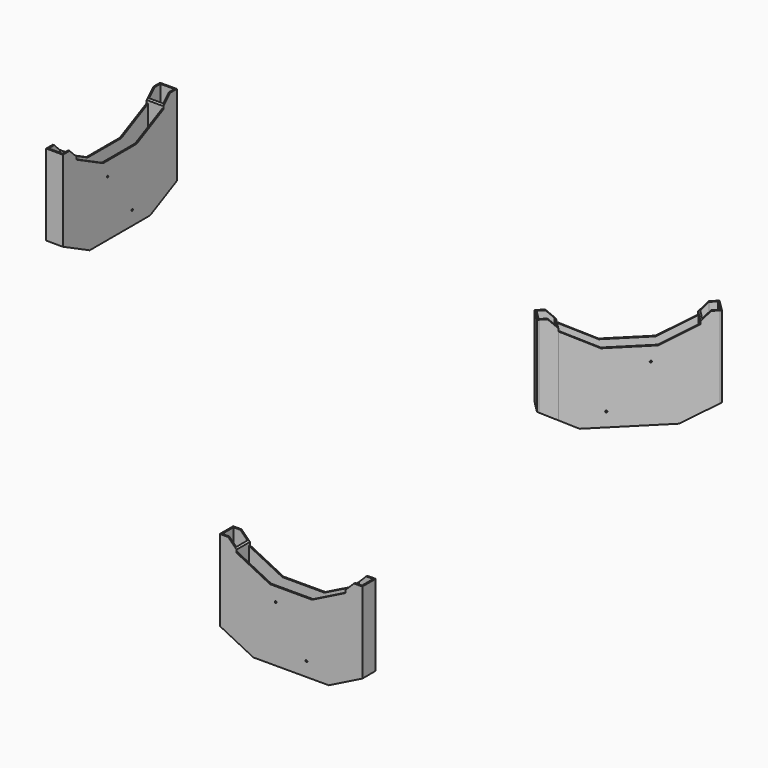
from build123d import *

# Parameters (mm, degrees)
F0_W          = 390
F0_H          = 5
F0_W_2        = 5
F0_H_2        = 50
F1_DEPTH      = 350
F0_H_3        = 390
F0_W_3        = 50
F2_R          = 3.25
F3_DEPTH      = 100
F4_R          = 3.25
F5_DEPTH      = 100
F6_R          = 3.25
F7_DEPTH      = 100
F8_T1_DEPTH   = 681.5589297088
F8_2_T1_DEPTH = 681.5589297088
F8_2_T3_DEPTH = 681.5589297088
F8_3_T1_DEPTH = 681.5589297088
F9_T1_DEPTH   = 214.3009792779
F9_2_T1_DEPTH = 214.300979278
F9_3_T1_DEPTH = 214.300979278


# Not quite as in the source:
# - a fillet or chamfer that OpenCascade refuses, or shapes differently, is made with other operations: its cross-section is extruded or revolved along the edge and cut away or added


with BuildPart() as f1:
    # F0 (on Top) → F1 (new body)
    with BuildSketch(Plane.XY):
        Polygon((90.3563703896, -1526.5155034513), (90.3563703896, -1531.5155034513), (480.3563703896, -1531.5155034513), (480.3563703896, -1526.5155034513), (460.3563703896, -1526.5155034513), (410.3563703896, -1526.5155034513), (160.3563703896, -1526.5155034513), (110.3563703896, -1526.5155034513), align=None)
        with Locations((285.3563703896, -1584.0155034513)):
            Rectangle(F0_W, F0_H)
        with Locations((87.8563703896, -1556.5155034513)):
            Rectangle(F0_W_2, F0_H_2)
        Polygon((30.3563703896, -1526.5155034513), (30.3563703896, -1531.5155034513), (35.3563703896, -1531.5155034513), (85.3563703896, -1531.5155034513), (90.3563703896, -1531.5155034513), (90.3563703896, -1526.5155034513), align=None)
        with Locations((32.8563703896, -1556.5155034513)):
            Rectangle(F0_W_2, F0_H_2)
        Polygon((30.3563703896, -1581.5155034513), (30.3563703896, -1586.5155034513), (90.3563703896, -1586.5155034513), (90.3563703896, -1581.5155034513), (85.3563703896, -1581.5155034513), (35.3563703896, -1581.5155034513), align=None)
        Polygon((480.3563703896, -1581.5155034513), (480.3563703896, -1586.5155034513), (540.3563703896, -1586.5155034513), (540.3563703896, -1581.5155034513), (535.3563703896, -1581.5155034513), (485.3563703896, -1581.5155034513), align=None)
        with Locations((482.8563703896, -1556.5155034513)):
            Rectangle(F0_W_2, F0_H_2)
        Polygon((480.3563703896, -1526.5155034513), (480.3563703896, -1531.5155034513), (485.3563703896, -1531.5155034513), (535.3563703896, -1531.5155034513), (540.3563703896, -1531.5155034513), (540.3563703896, -1526.5155034513), align=None)
        with Locations((537.8563703896, -1556.5155034513)):
            Rectangle(F0_W_2, F0_H_2)
    extrude(amount=F1_DEPTH)

    # F6 (on face) → F7 (cut)
    with BuildSketch(Plane.XZ.offset(1586.5155034513)):
        with Locations((230.3563703896, 200)):
            Circle(F6_R)
        with Locations((340.3563703896, 50)):
            Circle(F6_R)
        Polygon((480.3563703896, 350), (90.3563703896, 350), (90.3563703896, 310), (210.3563703896, 250), (360.3563703896, 250), (480.3563703896, 310), align=None)
    extrude(amount=-F7_DEPTH, mode=Mode.SUBTRACT)

    # F8: chamfer of 60 x 120 on 2 edges, made by hand

    # F8_s2 → F8_t1 (cut)
    with BuildSketch(Plane.XZ.offset(1215.7360385969)):
        Polygon((540.3563703896, 60), (420.3563703896, 0), (540.3563703896, 0), align=None)
        Polygon((30.3563703896, 60), (150.3563703896, 0), (30.3563703896, 0), align=None)
    extrude(amount=F8_T1_DEPTH, mode=Mode.SUBTRACT)

    # F9: chamfer of 30 on 2 edges, made by hand

    # F9_s2 → F9_t1 (cut)
    with BuildSketch(Plane.XZ.offset(1449.3650138123)):
        Polygon((510.3563703896, 350), (480.3563703896, 320), (480.3563703896, 350), align=None)
        Polygon((60.3563703896, 350), (90.3563703896, 320), (90.3563703896, 350), align=None)
    extrude(amount=F9_T1_DEPTH, mode=Mode.SUBTRACT)


with BuildPart() as f1b:
    # F0 (on Top) → F1, piece 2 (new body)
    with BuildSketch(Plane.XY):
        Polygon((215.6097792881, 288.056401427), (219.145313194, 284.520867521), (222.6808471, 288.056401427), (219.145313194, 291.5919353329), align=None)
        Polygon((197.9321097584, 270.3787318973), (201.4676436644, 266.8431979914), (219.145313194, 284.520867521), (215.6097792881, 288.056401427), align=None)
        Polygon((176.7189063228, 326.9472743922), (159.0412367932, 309.2696048626), (162.5767706991, 305.7340709566), (180.2544402288, 323.4117404863), align=None)
        Polygon((180.2544402288, 330.4828082982), (176.7189063228, 326.9472743922), (180.2544402288, 323.4117404863), (183.7899741347, 326.9472743922), align=None)
        Polygon((-44.251962798, 21.1235915291), (201.4676436644, 266.8431979914), (197.9321097584, 270.3787318973), (-47.7874967039, 24.659125435), align=None)
        Polygon((162.5767706991, 305.7340709566), (159.0412367932, 309.2696048626), (-86.6783696692, 63.5499984002), (-83.1428357632, 60.0144644943), align=None)
        Polygon((196.1643428055, 346.3927108749), (180.2544402288, 330.4828082982), (183.7899741347, 326.9472743922), (199.6998767114, 342.8571769689), align=None)
        Polygon((219.145313194, 291.5919353329), (222.6808471, 288.056401427), (238.5907496767, 303.9663040037), (235.0552157707, 307.5018379096), align=None)
        Polygon((-47.7874967039, 24.659125435), (-83.1428357632, 60.0144644943), (-86.6783696692, 56.4789305884), (-51.3230306098, 21.123591529), align=None)
        Polygon((-86.6783696692, 63.5499984002), (-125.5692426344, 24.659125435), (-122.0337087285, 21.123591529), (-86.6783696692, 56.4789305884), (-83.1428357632, 60.0144644943), align=None)
        Polygon((-122.0337087285, 21.123591529), (-125.5692426344, 17.5880576231), (-90.2139035751, -17.7672814362), (-86.6783696692, -14.2317475303), align=None)
        Polygon((-125.5692426344, 24.659125435), (-129.1047765404, 21.123591529), (-125.5692426344, 17.5880576231), (-122.0337087285, 21.123591529), align=None)
        Polygon((-90.2139035751, -17.7672814362), (-86.6783696692, -21.3028153421), (-83.1428357632, -17.7672814362), (-86.6783696692, -14.2317475303), align=None)
        Polygon((-86.6783696692, -14.2317475303), (-83.1428357632, -17.7672814362), (-44.251962798, 21.1235915291), (-47.7874967039, 24.659125435), (-51.3230306098, 21.123591529), align=None)
        Polygon((235.0552157707, 385.2835838401), (196.1643428055, 346.3927108749), (199.6998767114, 342.8571769689), (203.2354106173, 346.3927108749), (220.913080147, 364.0703804045), (238.5907496767, 381.7480499342), align=None)
        Polygon((203.2354106173, 346.3927108749), (199.6998767114, 342.8571769689), (235.0552157707, 307.5018379096), (238.5907496767, 311.0373718155), align=None)
        Polygon((235.0552157707, 307.5018379096), (238.5907496767, 303.9663040037), (277.4816226419, 342.8571769689), (273.946088736, 346.3927108749), (256.2684192063, 328.7150413452), (238.5907496767, 311.0373718155), align=None)
        Polygon((273.946088736, 346.3927108749), (277.4816226419, 342.8571769689), (281.0171565478, 346.3927108749), (277.4816226419, 349.9282447808), align=None)
        Polygon((242.1262835826, 385.2835838401), (238.5907496767, 381.7480499342), (273.946088736, 346.3927108749), (277.4816226419, 349.9282447808), align=None)
        Polygon((238.5907496767, 388.8191177461), (235.0552157707, 385.2835838401), (238.5907496767, 381.7480499342), (242.1262835826, 385.2835838401), align=None)
    extrude(amount=F1_DEPTH)

    # F2 (on face) → F3 (cut)
    with BuildSketch(Plane(origin=(-32.6877771635, 32.6877771635, 0), x_dir=(0.7071067812, 0.7071067812, 0), z_dir=(0.7071067812, -0.7071067812, 0))):
        with Locations((118.6457718379, 50)):
            Circle(F2_R)
        with Locations((243.6457718379, 200)):
            Circle(F2_R)
        Polygon((383.6457718379, 350), (-16.3542281621, 350), (-16.3542281621, 310), (103.6457718379, 250), (263.6457718379, 250), (383.6457718379, 310), align=None)
    extrude(amount=-F3_DEPTH, mode=Mode.SUBTRACT)

    # F8#2: chamfer of 60 x 120 on 2 edges, made by hand

    # F8_2_s2 → F8_2_t1 (cut)
    with BuildSketch(Plane(origin=(187.0664898886, -187.0664898886, 0), x_dir=(0, 0, 1), z_dir=(-0.7071067812, 0.7071067812, 0))):
        Polygon((60, 443.6457718379), (0, 323.6457718379), (0, 443.6457718379), align=None)
    extrude(amount=F8_2_T1_DEPTH, mode=Mode.SUBTRACT)

    # F8_2_s4 → F8_2_t3 (cut)
    with BuildSketch(Plane(origin=(-294.8684510868, 294.8684510868, 0), x_dir=(0, 0, 1), z_dir=(0.7071067812, -0.7071067812, 0))):
        Polygon((60, 76.3542281621), (0, -43.6457718379), (0, 76.3542281621), align=None)
    extrude(amount=F8_2_T3_DEPTH, mode=Mode.SUBTRACT)

    # F9#2: chamfer of 30 on 2 edges, made by hand

    # F9_2_s2 → F9_2_t1 (cut)
    with BuildSketch(Plane(origin=(-129.6678184303, 129.6678184303, 0), x_dir=(0, 0, 1), z_dir=(0.7071067812, -0.7071067812, 0))):
        Polygon((350, 46.3542281621), (320, 16.3542281621), (350, 16.3542281621), align=None)
        Polygon((350, -413.6457718379), (320, -383.6457718379), (350, -383.6457718379), align=None)
    extrude(amount=F9_2_T1_DEPTH, mode=Mode.SUBTRACT)


with BuildPart() as f1c:
    # F0 (on Top) → F1, piece 3 (new body)
    with BuildSketch(Plane.XY):
        Polygon((-1745.7581393137, -8.4296195955), (-1745.7581393137, 11.5703804045), (-1745.7581393137, 49.0703804045), (-1745.7581393137, 61.5703804045), (-1745.7581393137, 311.5703804045), (-1745.7581393137, 324.0703804045), (-1745.7581393137, 349.0703804045), (-1745.7581393137, 361.5703804045), (-1745.7581393137, 381.5703804045), (-1750.7581393137, 381.5703804045), (-1750.7581393137, -8.4296195955), align=None)
        with Locations((-1803.2581393137, 186.5703804045)):
            Rectangle(F0_W_2, F0_H_3)
        Polygon((-1805.7581393137, 381.5703804045), (-1800.7581393137, 381.5703804045), (-1800.7581393137, 386.5703804045), (-1800.7581393137, 436.5703804045), (-1800.7581393137, 441.5703804045), (-1805.7581393137, 441.5703804045), align=None)
        with Locations((-1775.7581393137, 439.0703804045)):
            Rectangle(F0_W_3, F0_H)
        Polygon((-1750.7581393137, 381.5703804045), (-1745.7581393137, 381.5703804045), (-1745.7581393137, 441.5703804045), (-1750.7581393137, 441.5703804045), (-1750.7581393137, 436.5703804045), (-1750.7581393137, 386.5703804045), align=None)
        with Locations((-1775.7581393137, 384.0703804045)):
            Rectangle(F0_W_3, F0_H)
        Polygon((-1800.7581393137, -13.4296195955), (-1800.7581393137, -8.4296195955), (-1805.7581393137, -8.4296195955), (-1805.7581393137, -63.4296195955), (-1800.7581393137, -63.4296195955), align=None)
        with Locations((-1775.7581393137, -10.9296195955)):
            Rectangle(F0_W_3, F0_H)
        Polygon((-1745.7581393137, -63.4296195955), (-1745.7581393137, -8.4296195955), (-1750.7581393137, -8.4296195955), (-1750.7581393137, -13.4296195955), (-1750.7581393137, -63.4296195955), align=None)
        with Locations((-1748.2581393137, -65.9296195955)):
            Rectangle(F0_W_2, F0_H)
        with Locations((-1775.7581393137, -65.9296195955)):
            Rectangle(F0_W_3, F0_H)
        with Locations((-1803.2581393137, -65.9296195955)):
            Rectangle(F0_W_2, F0_H)
    extrude(amount=F1_DEPTH)

    # F4 (on face) → F5 (cut)
    with BuildSketch(Plane.YZ.offset(-1745.7581393137)):
        with Locations((131.5703804045, 200)):
            Circle(F4_R)
        with Locations((241.5703804045, 50)):
            Circle(F4_R)
        Polygon((381.5703804045, 310), (381.5703804045, 350), (-8.4296195955, 350), (-8.4296195955, 310), (111.5703804045, 250), (261.5703804045, 250), align=None)
    extrude(amount=-F5_DEPTH, mode=Mode.SUBTRACT)

    # F8#3: chamfer of 60 x 120 on 2 edges, made by hand

    # F8_3_s2 → F8_3_t1 (cut)
    with BuildSketch(Plane.YZ.offset(-2116.5376041681)):
        Polygon((441.5703804045, 60), (321.5703804045, 0), (441.5703804045, 0), align=None)
        Polygon((-68.4296195955, 60), (51.5703804045, 0), (-68.4296195955, 0), align=None)
    extrude(amount=F8_3_T1_DEPTH, mode=Mode.SUBTRACT)

    # F9#3: chamfer of 30 on 2 edges, made by hand

    # F9_3_s2 → F9_3_t1 (cut)
    with BuildSketch(Plane.YZ.offset(-1882.9086289527)):
        Polygon((-38.4296195955, 350), (-8.4296195955, 320), (-8.4296195955, 350), align=None)
        Polygon((381.5703804045, 320), (411.5703804045, 350), (381.5703804045, 350), align=None)
    extrude(amount=F9_3_T1_DEPTH, mode=Mode.SUBTRACT)


solid = Compound([f1.part, f1b.part, f1c.part])
